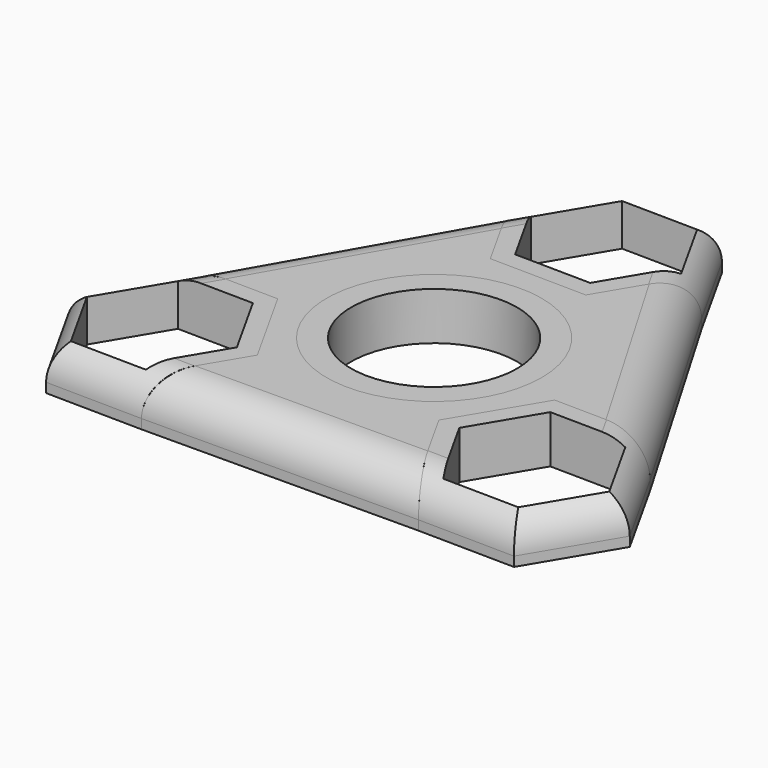
from build123d import *

# Parameters (mm, degrees)
F1_R          = 14.2875
F2_DEPTH      = 6.35
F0_R          = 14.2875
F0_R_2        = 11.0236
F3_T1_DEPTH   = 38.2316097327
F3_T3_DEPTH   = 38.2316097327
F3_T5_DEPTH   = 38.2316097327
F3_2_F1_R     = 5.08
F3_2_F2_R     = 5.08
F3_2_F3_R     = 5.08
F3_3_T1_DEPTH = 38.2316097327
F3_3_T3_DEPTH = 38.2316097327
F3_3_T5_DEPTH = 38.2316097327
F3_4_T1_DEPTH = 38.2316097327
F3_4_T3_DEPTH = 38.2316097327
F3_4_T5_DEPTH = 38.2316097327


# Not quite as in the source:
# - a fillet or chamfer that OpenCascade refuses, or shapes differently, is made with other operations: its cross-section is extruded or revolved along the edge and cut away or added


with BuildPart() as f2:
    # F1 (on Top) → F2 (new body)
    with BuildSketch(Plane.XY):
        Polygon((12.8303093344, 28.3923234629), (9.543630774, 22.8823057434), (6.2569521454, 17.3722879094), (-0.1582021818, 17.4636261732), (-6.573357189, 17.5549644466), (-9.7018333012, 23.1563205626), (-12.8303093344, 28.7576765371), (-31.0036280585, -3.0847879094), (-24.5884733182, -3.176126179), (-18.1733187241, -3.2674644466), (-15.0448426119, -8.8688205626), (-11.9163665788, -14.4701765371), (-15.2030451391, -19.9801942566), (-18.4897237678, -25.4902120906), (18.1733187241, -25.3075355534), (15.0448429163, -19.7061799824), (11.9163665788, -14.1048234629), (15.2030453836, -8.5948053335), (18.4897237678, -3.0847879094), (24.9048784863, -3.1761261787), (31.3200331022, -3.2674644466), align=None)
        Circle(F1_R, mode=Mode.SUBTRACT)
    extrude(amount=F2_DEPTH)

    # F3#2: fillet of radius 5.08 on 3 edges, made by hand

    # F3_2_f1
    f3_2_f1_edges = [f2.edges().sort_by_distance(p)[0] for p in [
        (-21.9169686964, 12.8364443138, 6.35),
    ]]
    fillet(f3_2_f1_edges, radius=F3_2_F1_R)

    # F3_2_f2
    f3_2_f2_edges = [f2.edges().sort_by_distance(p)[0] for p in [
        (22.0751712183, 12.5624295081, 6.35),
    ]]
    fillet(f3_2_f2_edges, radius=F3_2_F2_R)

    # F3_2_f3
    f3_2_f3_edges = [f2.edges().sort_by_distance(p)[0] for p in [
        (-0.1582025218, -25.398873822, 6.35),
    ]]
    fillet(f3_2_f3_edges, radius=F3_2_F3_R)


with BuildPart() as f2b:
    # F0 (on Top) → F2, piece 2 (new body)
    with BuildSketch(Plane.XY):
        Polygon((6.2569521454, 17.3722879094), (12.8303093344, 28.3923234629), (6.573357189, 39.5950355534), (-6.2569521454, 39.7777120906), (-12.8303093344, 28.7576765371), (-6.573357189, 17.5549644466), align=None)
        Polygon((5.1647806485, 37.2335993634), (10.0809573342, 28.4314684351), (4.9161766856, 19.7728690717), (-5.1647806485, 19.9164006366), (-10.0809573342, 28.7185315649), (-4.9161766856, 37.3771309283), align=None, mode=Mode.SUBTRACT)
    extrude(amount=F2_DEPTH)

    # F3: fillet of radius 5.08 on 3 edges, made by hand

    # F3_s2 → F3_t1 (cut)
    with BuildSketch(Plane(origin=(22.3643199705, 37.4931095506, 0), x_dir=(0, 0, 1), z_dir=(-0.5122784534, -0.8588194142, 0))):
        with BuildLine():
            ThreePointArc((1.27, 25.750856807), (4.8621024484, 24.2629592555), (6.35, 20.670856807))
            Line((6.35, 20.670856807), (6.35, 25.750856807))
            Line((6.35, 25.750856807), (1.27, 25.750856807))
        make_face()
    extrude(amount=F3_T1_DEPTH, mode=Mode.SUBTRACT)

    # F3_s4 → F3_t3 (cut)
    with BuildSketch(Plane(origin=(-2.8436871063, 5.0914578197, 0), x_dir=(0, 0, 1), z_dir=(-0.4876202032, 0.8730558616, 0))):
        with BuildLine():
            ThreePointArc((1.27, 25.0462473067), (4.8621024484, 23.5583497551), (6.35, 19.9662473067))
            Line((6.35, 19.9662473067), (6.35, 25.0462473067))
            Line((6.35, 25.0462473067), (1.27, 25.0462473067))
        make_face()
    extrude(amount=F3_T3_DEPTH, mode=Mode.SUBTRACT)

    # F3_s6 → F3_t5 (cut)
    with BuildSketch(Plane(origin=(18.707102349, -0.2663496715, 0), x_dir=(0, 0, 1), z_dir=(-0.9998986566, 0.0142364474, 0))):
        with BuildLine():
            ThreePointArc((1.27, 39.6846041137), (4.8621024484, 38.1967065621), (6.35, 34.6046041137))
            Line((6.35, 34.6046041137), (6.35, 39.6846041137))
            Line((6.35, 39.6846041137), (1.27, 39.6846041137))
        make_face()
    extrude(amount=F3_T5_DEPTH, mode=Mode.SUBTRACT)


with BuildPart() as f2c:
    # F0 (on Top) → F2, piece 3 (new body)
    with BuildSketch(Plane.XY):
        Circle(F0_R)
        Circle(F0_R_2, mode=Mode.SUBTRACT)
    extrude(amount=F2_DEPTH)


with BuildPart() as f2d:
    # F0 (on Top) → F2, piece 4 (new body)
    with BuildSketch(Plane.XY):
        Polygon((18.4897237678, -3.0847879094), (11.9163665788, -14.1048234629), (18.1733187241, -25.3075355534), (31.0036280585, -25.4902120906), (37.5769852475, -14.4701765371), (31.3200331022, -3.2674644466), align=None)
        Polygon((19.5818952646, -22.9460993634), (14.665718579, -14.1439684351), (19.8304992275, -5.4853690717), (29.9114565617, -5.6289006366), (34.8276332473, -14.4310315649), (29.6628525988, -23.0896309283), align=None, mode=Mode.SUBTRACT)
    extrude(amount=F2_DEPTH)

    # F3#4: fillet of radius 5.08 on 3 edges, made by hand

    # F3_4_s2 → F3_4_t1 (cut)
    with BuildSketch(Plane(origin=(5.8311753673, -0.0830236353, 0), x_dir=(0, 0, 1), z_dir=(0.9998986566, -0.0142364474, 0))):
        with BuildLine():
            ThreePointArc((1.27, 25.0462473067), (4.8621024484, 23.5583497551), (6.35, 19.9662473067))
            Line((6.35, 19.9662473067), (6.35, 25.0462473067))
            Line((6.35, 25.0462473067), (1.27, 25.0462473067))
        make_face()
    extrude(amount=F3_4_T1_DEPTH, mode=Mode.SUBTRACT)

    # F3_4_s4 → F3_4_t3 (cut)
    with BuildSketch(Plane(origin=(-9.5842167564, -16.0676510297, 0), x_dir=(0, 0, 1), z_dir=(0.5122784534, 0.8588194142, 0))):
        with BuildLine():
            ThreePointArc((1.27, 39.6846041137), (4.8621024484, 38.1967065621), (6.35, 34.6046041137))
            Line((6.35, 34.6046041137), (6.35, 39.6846041137))
            Line((6.35, 39.6846041137), (1.27, 39.6846041137))
        make_face()
    extrude(amount=F3_4_T3_DEPTH, mode=Mode.SUBTRACT)

    # F3_4_s6 → F3_4_t5 (cut)
    with BuildSketch(Plane(origin=(21.2878253524, -38.1146240081, 0), x_dir=(0, 0, 1), z_dir=(-0.4876202032, 0.8730558616, 0))):
        with BuildLine():
            ThreePointArc((1.27, 25.750856807), (4.8621024484, 24.2629592555), (6.35, 20.670856807))
            Line((6.35, 20.670856807), (6.35, 25.750856807))
            Line((6.35, 25.750856807), (1.27, 25.750856807))
        make_face()
    extrude(amount=F3_4_T5_DEPTH, mode=Mode.SUBTRACT)


with BuildPart() as f2e:
    # F0 (on Top) → F2, piece 5 (new body)
    with BuildSketch(Plane.XY):
        Polygon((-11.9163665788, -14.4701765371), (-18.1733187241, -3.2674644466), (-31.0036280585, -3.0847879094), (-37.5769852475, -14.1048234629), (-31.3200331022, -25.3075355534), (-18.4897237678, -25.4902120906), align=None)
        Polygon((-29.6628525988, -5.4853690717), (-19.5818952646, -5.6289006366), (-14.665718579, -14.4310315649), (-19.8304992275, -23.0896309283), (-29.9114565617, -22.9460993634), (-34.8276332473, -14.1439684351), align=None, mode=Mode.SUBTRACT)
    extrude(amount=F2_DEPTH)

    # F3#3: fillet of radius 5.08 on 3 edges, made by hand

    # F3_3_s2 → F3_3_t1 (cut)
    with BuildSketch(Plane(origin=(-2.987488261, -5.0084341843, 0), x_dir=(0, 0, 1), z_dir=(-0.5122784534, -0.8588194142, 0))):
        with BuildLine():
            ThreePointArc((1.27, 25.0462473067), (4.8621024484, 23.5583497551), (6.35, 19.9662473067))
            Line((6.35, 19.9662473067), (6.35, 25.0462473067))
            Line((6.35, 25.0462473067), (1.27, 25.0462473067))
        make_face()
    extrude(amount=F3_3_T1_DEPTH, mode=Mode.SUBTRACT)

    # F3_3_s4 → F3_3_t3 (cut)
    with BuildSketch(Plane(origin=(-9.1228855927, 16.3340007012, 0), x_dir=(0, 0, 1), z_dir=(0.4876202032, -0.8730558616, 0))):
        with BuildLine():
            ThreePointArc((1.27, 39.6846041137), (4.8621024484, 38.1967065621), (6.35, 34.6046041137))
            Line((6.35, 34.6046041137), (6.35, 39.6846041137))
            Line((6.35, 39.6846041137), (1.27, 39.6846041137))
        make_face()
    extrude(amount=F3_3_T3_DEPTH, mode=Mode.SUBTRACT)

    # F3_3_s6 → F3_3_t5 (cut)
    with BuildSketch(Plane(origin=(-43.6521453229, 0.6215144576, 0), x_dir=(0, 0, 1), z_dir=(0.9998986566, -0.0142364474, 0))):
        with BuildLine():
            ThreePointArc((1.27, 25.750856807), (4.8621024484, 24.2629592555), (6.35, 20.670856807))
            Line((6.35, 20.670856807), (6.35, 25.750856807))
            Line((6.35, 25.750856807), (1.27, 25.750856807))
        make_face()
    extrude(amount=F3_3_T5_DEPTH, mode=Mode.SUBTRACT)


solid = Compound([f2.part, f2b.part, f2c.part, f2d.part, f2e.part])
